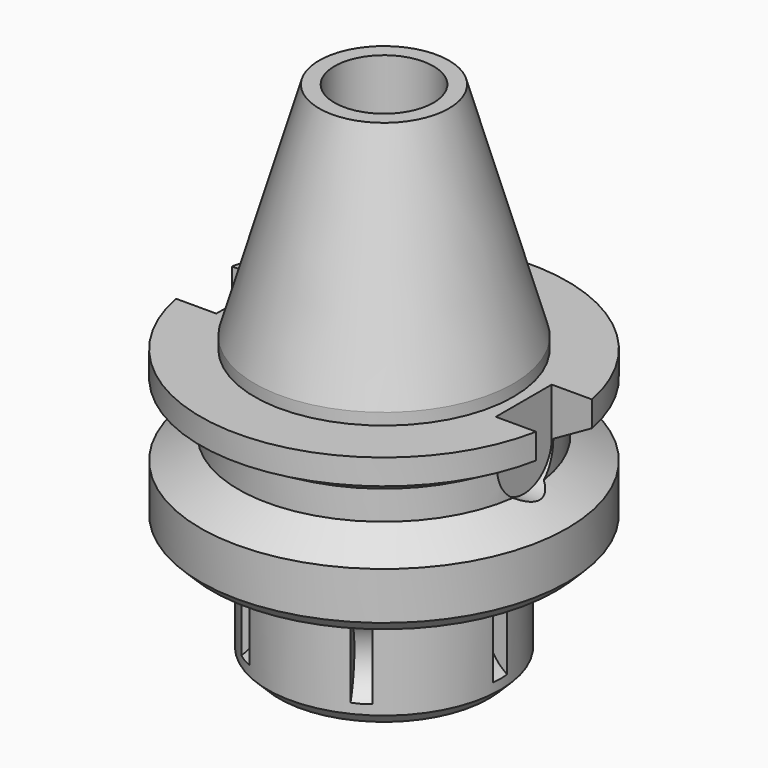
from build123d import *

# Parameters (mm, degrees)
F0_W            = 25
F0_H            = 4.9944465005
F0_W_2          = 20
F0_H_2          = 20
F2_SIZE         = 2
F5_DEPTH        = 63.5294467211
F7_R            = 7.5
F8_DEPTH        = 1.5
F8_COPIES_COUNT = 6
F9_R            = 8.5
F10_DEPTH       = 89.8396968842


# Not quite as in the source:
# - a pattern or mirror of a feature is missing from the dataset's text; its kind, count and spacing are read off the source's solid


with BuildPart() as f1:
    # F0 (on Front) → F1 (revolve)
    with BuildSketch(Plane.XZ):
        Polygon((0, 40), (0, 0), (22.225, 0), (22.225, 2), (11.1490100557, 40), align=None)
        Polygon((22.225, 0), (0, 0), (0, -4.35), (31.5, -4.35), (31.5, 0), align=None)
        Polygon((31.5, -4.35), (0, -4.35), (0, -8.1027767497), (25, -8.1027767497), align=None)
        with Locations((12.5, -10.6)):
            Rectangle(F0_W, F0_H)
        Polygon((25, -13.0972232503), (0, -13.0972232503), (0, -16.85), (31.5, -16.85), align=None)
        Polygon((31.5, -16.85), (0, -16.85), (0, -27), (20, -27), (31.5, -27), align=None)
        with Locations((10, -37)):
            Rectangle(F0_W_2, F0_H_2)
    revolve(axis=Axis((0, 0, -0.6091467625), (0, 0, -1)))

    # F2
    f2_edges = [f1.edges().sort_by_distance(p)[0] for p in [
        (-31.5, 0, -27),
        (-20, 0, -47),
    ]]
    chamfer(f2_edges, length=F2_SIZE)

    # F4 (on offset) → F5 (cut)
    with BuildSketch(Plane.YZ.offset(24)):
        with BuildLine():
            ThreePointArc((-6, -8.1027767497), (0, -14.1027767497), (6, -8.1027767497))
            ThreePointArc((6, -8.1027767497), (0, -2.1027767497), (-6, -8.1027767497))
        make_face()
        with BuildLine():
            ThreePointArc((-6, -8.1027767497), (0, -2.1027767497), (6, -8.1027767497))
            Line((6, -8.1027767497), (6, 0))
            Line((6, 0), (-6, 0))
            Line((-6, 0), (-6, -8.1027767497))
        make_face()
    extrude(amount=F5_DEPTH, mode=Mode.SUBTRACT)

    # F6: F1 across plane


with BuildPart() as f1_1:
    add(f1.part)
    add(f1.part.mirror(Plane.YZ), mode=Mode.INTERSECT)

    # F7 (on Front) → F8 (cut, symmetric)
    with BuildSketch(Plane.XZ):
        with Locations((24, -37)):
            Circle(F7_R)
    f8 = extrude(amount=F8_DEPTH, both=True, mode=Mode.SUBTRACT)

    # F8_copies: F8 ×6 about axis
    f8_copies_axis = Axis((0, 0, 0), (0, 0, 1))
    for i in range(1, F8_COPIES_COUNT):
        add(f8.rotate(f8_copies_axis, i * 360 / F8_COPIES_COUNT), mode=Mode.SUBTRACT)

    # F9 (on Top) → F10 (cut)
    with BuildSketch(Plane.XY):
        Circle(F9_R)
    extrude(amount=F10_DEPTH, mode=Mode.SUBTRACT)


solid = f1_1.part
